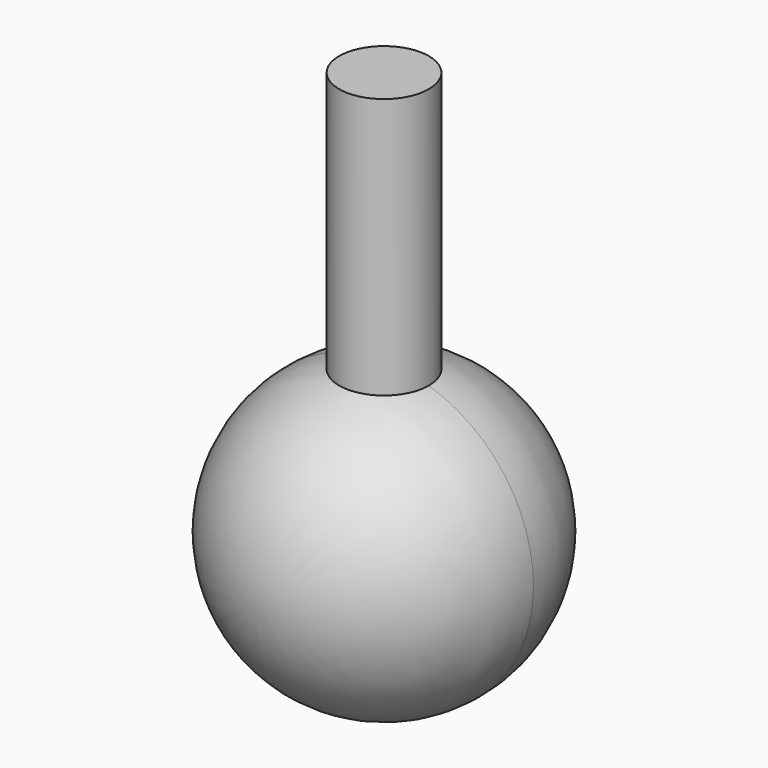
from build123d import *

# Parameters (mm, degrees)
F0_R     = 50
F1_DEPTH = 50
F2_R     = 49.99999
F3_R     = 15
F4_DEPTH = 135


# Not quite as in the source:
# - a fillet or chamfer is up to 0.001 mm smaller than in the source, because OpenCascade refuses the exact size


with BuildPart() as f1:
    # F0 (on Front) → F1 (new body, symmetric)
    with BuildSketch(Plane.XZ):
        Circle(F0_R)
    extrude(amount=F1_DEPTH, both=True)

    # F2 (radius 50 in the source; OpenCascade refuses exactly that, so slightly less here)
    f2_edges = [f1.edges().sort_by_distance(p)[0] for p in [
        (-50, -50, 0),
        (-50, 50, 0),
    ]]
    fillet(f2_edges, radius=F2_R)

    # F3 (on Top) → F4 (join)
    with BuildSketch(Plane.XY):
        Circle(F3_R)
    extrude(amount=F4_DEPTH)


solid = f1.part
